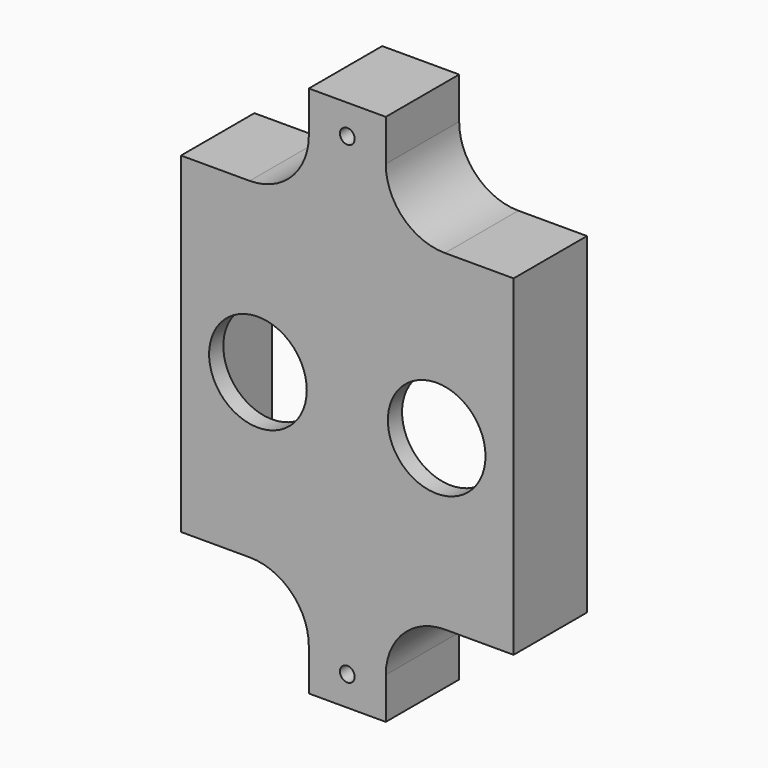
from build123d import *

# Parameters (mm, degrees)
F0_W        = 56.2
F0_H        = 56
F0_W_2      = 50.2
F0_H_2      = 50
F0_R        = 8.25
F1_DEPTH    = 3
F2_DEPTH    = 12.5
F3_W        = 13
F3_H        = 17
F3_R        = 1.25
F4_DEPTH    = 15.5
F5_R        = 10
F6_T        = 3
F6_T3_DEPTH = 56.2
F6_T5_DEPTH = 56
F6_T7_DEPTH = 18.5


# Not quite as in the source:
# - a shell that OpenCascade refuses in one call is made with other operations: the cavity is built on its own and cut out


with BuildPart() as f1:
    # F0 (on Front) → F1 (new body)
    with BuildSketch(Plane.XZ):
        Rectangle(F0_W, F0_H)
        Rectangle(F0_W_2, F0_H_2, mode=Mode.SUBTRACT)
        Rectangle(F0_W_2, F0_H_2)
        with Locations((-15.1, 0)):
            Circle(F0_R, mode=Mode.SUBTRACT)
        with Locations((15.1, 0)):
            Circle(F0_R, mode=Mode.SUBTRACT)
    extrude(amount=F1_DEPTH)

    # F0 (on Front) → F2 (join)
    with BuildSketch(Plane.XZ):
        Rectangle(F0_W, F0_H)
        Rectangle(F0_W_2, F0_H_2, mode=Mode.SUBTRACT)
    extrude(amount=-F2_DEPTH)

    # F3 (on face) → F4 (join, through all)
    with BuildSketch(Plane.XZ.offset(3)):
        with Locations((0, 36.5)):
            Rectangle(F3_W, F3_H)
        with Locations((0, 40)):
            Circle(F3_R, mode=Mode.SUBTRACT)
        with Locations((0, -36.5)):
            Rectangle(F3_W, F3_H)
        with Locations((0, -40)):
            Circle(F3_R, mode=Mode.SUBTRACT)
    extrude(amount=-F4_DEPTH)

    # F5
    f5_edges = [f1.edges().sort_by_distance(p)[0] for p in [
        (6.5, 4.75, -28),
        (-6.5, 4.75, -28),
        (-6.5, 4.75, 28),
        (6.5, 4.75, 28),
    ]]
    fillet(f5_edges, radius=F5_R)

    # F6: shell of thickness 3, made by hand


with BuildPart() as f6_core1:
    # F6_t2: copy of F1
    add(f1.part)

    # the walls: a layer under each face that stays
    f6_faces = [f6_core1.faces().sort_by_distance(p)[0] for p in [
        (0, -3, 0),
        (22.3, 4.75, 28),
        (9.4289321881, 4.75, 30.9289321881),
        (28.1, 4.75, 0),
        (6.5, 4.75, 41.5),
        (22.3, 4.75, -28),
        (0, 4.75, 45),
        (9.4289321881, 4.75, -30.9289321881),
        (-6.5, 4.75, 41.5),
        (6.5, 4.75, -41.5),
        (-9.4289321881, 4.75, 30.9289321881),
        (0, 4.75, -45),
        (-22.3, 4.75, 28),
        (-6.5, 4.75, -41.5),
        (-28.1, 4.75, 0),
        (-9.4289321881, 4.75, -30.9289321881),
        (-22.3, 4.75, -28),
        (-23.35, -1.5, 0),
        (6.85, -1.5, 0),
        (-1.25, 4.75, 40),
        (-1.25, 4.75, -40),
        (0, 0, 0),
        (0, 6.25, 25),
        (25.1, 6.25, 0),
        (0, 6.25, -25),
        (-25.1, 6.25, 0),
    ]]
    thicken(f6_faces, amount=-F6_T, mode=Mode.SUBTRACT)

    # F6_s4 → F6_t3 (cut)
    with BuildSketch(Plane.YZ.offset(-28.1)):
        Polygon((0.03, 24.97), (-3, 25), (-3, 28), (0, 28), align=None)
        Polygon((0.03, -24.97), (-3, -25), (-3, -28), (0, -28), align=None)
    extrude(amount=F6_T3_DEPTH, mode=Mode.SUBTRACT)

    # F6_s6 → F6_t5 (cut)
    with BuildSketch(Plane.XY.offset(-28)):
        Polygon((25.07, 0.03), (25.1, -3), (28.1, -3), (28.1, 0), align=None)
        Polygon((-25.07, 0.03), (-25.1, -3), (-28.1, -3), (-28.1, 0), align=None)
    extrude(amount=F6_T5_DEPTH, mode=Mode.SUBTRACT)

    # F6_s8 → F6_t7 (cut)
    with BuildSketch(Plane.XZ.offset(-15.5)):
        Polygon((-25.07, 24.97), (-25.1, 28), (-28.1, 28), (-28.1, 25), align=None)
        Polygon((25.07, 24.97), (25.1, 28), (28.1, 28), (28.1, 25), align=None)
        Polygon((25.07, -24.97), (28.1, -25), (28.1, -28), (25.1, -28), align=None)
        Polygon((-25.07, -24.97), (-25.1, -28), (-28.1, -28), (-28.1, -25), align=None)
    extrude(amount=F6_T7_DEPTH, mode=Mode.SUBTRACT)


with BuildPart() as f1_1:
    add(f1.part)

    # what is left inside the walls is the cavity
    f6_cavity = [f6_core1.part.solids().sort_by_distance(p)[0] for p in [
        (0, 8.333333, 28.03),
        (0, 8.333333, -28.03),
    ]]
    add(f6_cavity, mode=Mode.SUBTRACT)


solid = f1_1.part
